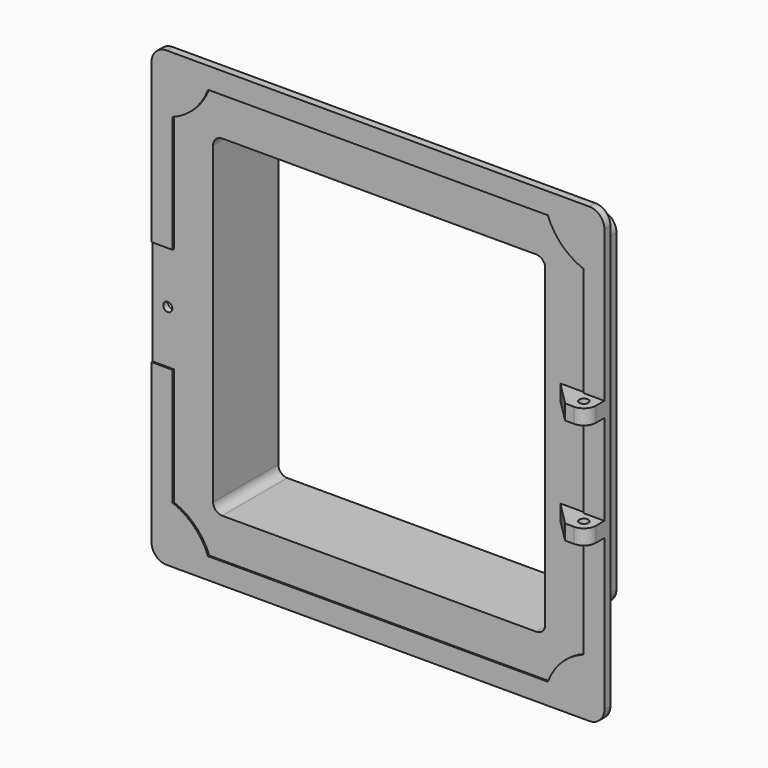
from build123d import *

# Parameters (mm, degrees)
F0_R     = 1.5
F0_W     = 114
F0_H     = 114
F0_W_2   = 110
F0_H_2   = 110
F1_DEPTH = 2
F0_W_3   = 7
F0_H_3   = 30
F2_DEPTH = 2.5
F0_H_4   = 5
F0_W_4   = 8
F3_DEPTH = 10
F4_SIZE  = 7.99999
F5_R     = 4
F6_DEPTH = 25
F7_R     = 3
F8_R     = 5
F10_D    = 3


# Not quite as in the source:
# - a fillet or chamfer is up to 0.001 mm smaller than in the source, because OpenCascade refuses the exact size


with BuildPart() as f1:
    # F0 (on Front) → F1 (new body)
    with BuildSketch(Plane.XZ):
        with BuildLine():
            Line((-68, 17.5), (-75, 17.5))
            Line((-75, 17.5), (-75, -17.5))
            Line((-75, -17.5), (-68, -17.5))
            Line((-68, -17.5), (-68, -56.2650060048))
            ThreePointArc((-68, -56.2650060048), (-60.8578643763, -60.8578643763), (-56.2650060048, -68))
            Line((-56.2650060048, -68), (56.2650060048, -68))
            ThreePointArc((56.2650060048, -68), (60.8578643763, -60.8578643763), (68, -56.2650060048))
            Line((68, -56.2650060048), (68, -20))
            Line((68, -20), (60, -20))
            Line((60, -20), (60, -15))
            Line((60, -15), (68, -15))
            Line((68, -15), (68, 15))
            Line((68, 15), (60, 15))
            Line((60, 15), (60, 20))
            Line((60, 20), (68, 20))
            Line((68, 20), (68, 56.2650060048))
            ThreePointArc((68, 56.2650060048), (60.8578643763, 60.8578643763), (56.2650060048, 68))
            Line((56.2650060048, 68), (-56.2650060048, 68))
            ThreePointArc((-56.2650060048, 68), (-60.8578643763, 60.8578643763), (-68, 56.2650060048))
            Line((-68, 56.2650060048), (-68, 17.5))
        make_face()
        with Locations((-70, 0)):
            Circle(F0_R, mode=Mode.SUBTRACT)
        Rectangle(F0_W, F0_H, mode=Mode.SUBTRACT)
        Rectangle(F0_W, F0_H)
        Rectangle(F0_W_2, F0_H_2, mode=Mode.SUBTRACT)
    extrude(amount=F1_DEPTH)

    # F0 (on Front) → F2 (join)
    with BuildSketch(Plane.XZ):
        with BuildLine():
            Line((-68, 68), (-68, 56.2650060048))
            ThreePointArc((-68, 56.2650060048), (-60.8578643763, 60.8578643763), (-56.2650060048, 68))
            Line((-56.2650060048, 68), (-68, 68))
        make_face()
        Polygon((75, 20), (75, 75), (-75, 75), (-75, 17.5), (-68, 17.5), (-68, 56.2650060048), (-68, 68), (-56.2650060048, 68), (56.2650060048, 68), (68, 68), (68, 56.2650060048), (68, 20), align=None)
        with BuildLine():
            ThreePointArc((56.2650060048, 68), (60.8578643763, 60.8578643763), (68, 56.2650060048))
            Line((68, 56.2650060048), (68, 68))
            Line((68, 68), (56.2650060048, 68))
        make_face()
        with BuildLine():
            Line((68, -68), (68, -56.2650060048))
            ThreePointArc((68, -56.2650060048), (60.8578643763, -60.8578643763), (56.2650060048, -68))
            Line((56.2650060048, -68), (68, -68))
        make_face()
        with BuildLine():
            ThreePointArc((-56.2650060048, -68), (-60.8578643763, -60.8578643763), (-68, -56.2650060048))
            Line((-68, -56.2650060048), (-68, -68))
            Line((-68, -68), (-56.2650060048, -68))
        make_face()
        Polygon((-68, -17.5), (-75, -17.5), (-75, -75), (75, -75), (75, -20), (68, -20), (68, -56.2650060048), (68, -68), (56.2650060048, -68), (-56.2650060048, -68), (-68, -68), (-68, -56.2650060048), align=None)
        with Locations((71.5, 0)):
            Rectangle(F0_W_3, F0_H_3)
    extrude(amount=F2_DEPTH)

    # F0 (on Front) → F3 (join)
    with BuildSketch(Plane.XZ):
        with Locations((71.5, 17.5)):
            Rectangle(F0_W_3, F0_H_4)
        with Locations((64, 17.5)):
            Rectangle(F0_W_4, F0_H_4)
        with Locations((64, -17.5)):
            Rectangle(F0_W_4, F0_H_4)
        with Locations((71.5, -17.5)):
            Rectangle(F0_W_3, F0_H_4)
    extrude(amount=F3_DEPTH)

    # F4 (size 8 in the source; OpenCascade refuses exactly that, so slightly less here)
    f4_edges = [f1.edges().sort_by_distance(p)[0] for p in [
        (60, -10, 17.5),
        (60, -10, -17.5),
    ]]
    chamfer(f4_edges, length=F4_SIZE)

    # F5
    f5_edges = [f1.edges().sort_by_distance(p)[0] for p in [
        (75, -10, 17.5),
        (75, -10, -17.5),
    ]]
    fillet(f5_edges, radius=F5_R)

    # F0 (on Front) → F6 (join)
    with BuildSketch(Plane.XZ):
        Rectangle(F0_W, F0_H)
        Rectangle(F0_W_2, F0_H_2, mode=Mode.SUBTRACT)
    extrude(amount=-F6_DEPTH)

    # F7
    f7_edges = [f1.edges().sort_by_distance(p)[0] for p in [
        (-55, 11.5, 55),
        (55, 11.5, 55),
        (55, 11.5, -55),
        (-55, 11.5, -55),
    ]]
    fillet(f7_edges, radius=F7_R)

    # F8
    f8_edges = [f1.edges().sort_by_distance(p)[0] for p in [
        (57, 12.5, 57),
        (57, 12.5, -57),
        (-57, 12.5, -57),
        (-57, 12.5, 57),
        (-75, -1.25, 75),
        (-75, -1.25, -75),
        (75, -1.25, -75),
        (75, -1.25, 75),
    ]]
    fillet(f8_edges, radius=F8_R)

    # F10 (through all)
    with Locations(Plane.XY.offset(20)):
        with Locations((71, -6)):
            Hole(F10_D / 2)


solid = f1.part
